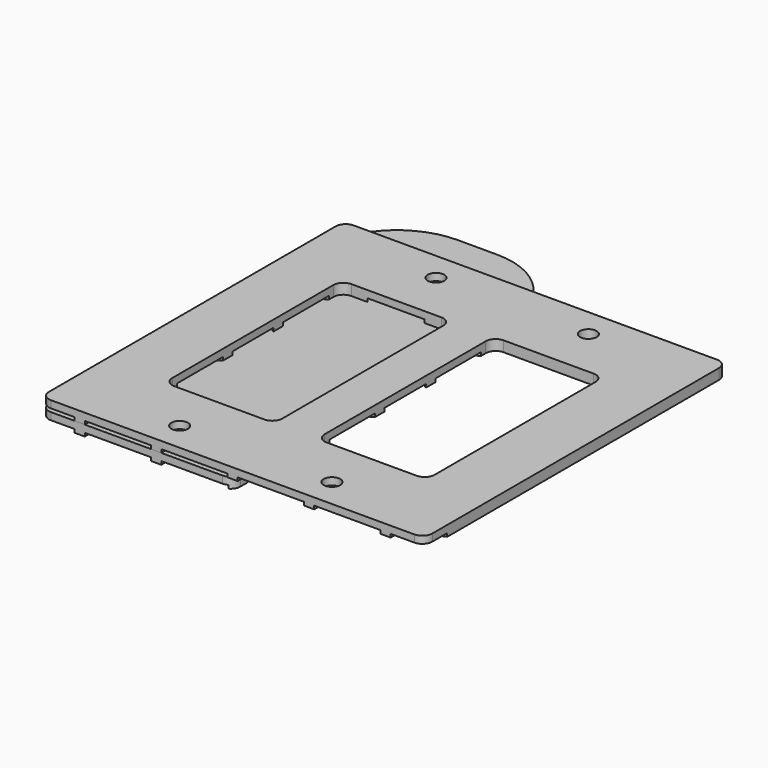
from build123d import *

# Parameters (mm, degrees)
F0_W     = 57.9
F0_H     = 114.3
F0_R     = 2.5
F0_W_2   = 33.2
F0_H_2   = 66.8
F1_DEPTH = 3.175
F2_R     = 2.5
F3_DEPTH = 3.175
F4_R     = 3
F4_2_R   = 3
F7_DEPTH = 1
F8_DEPTH = 4.175


# Not quite as in the source:
# - a length typed as a fraction of an inch, garbled in the dataset ("3 / 203.2 mm" for 3/8 in), is restored


with BuildPart() as f1:
    # F0 (on Top) → F1 (new body)
    with BuildSketch(Plane.XY):
        with Locations((-28.95, 0)):
            Rectangle(F0_W, F0_H)
        with Locations((-23, -48.4)):
            Circle(F0_R, mode=Mode.SUBTRACT)
        with Locations((-23, 0)):
            Rectangle(F0_W_2, F0_H_2, mode=Mode.SUBTRACT)
        with Locations((-23, 48.4)):
            Circle(F0_R, mode=Mode.SUBTRACT)
    extrude(amount=F1_DEPTH)

    # F4
    f4_edges = [f1.edges().sort_by_distance(p)[0] for p in [
        (-57.9, 57.15, 1.5875),
        (-57.9, -57.15, 1.5875),
        (-39.6, 33.4, 1.5875),
        (-39.6, -33.4, 1.5875),
        (-6.4, -33.4, 1.5875),
        (-6.4, 33.4, 1.5875),
    ]]
    fillet(f4_edges, radius=F4_R)

    # F5: F1 across face


with BuildPart() as f3:
    # F2 (on Top) → F3 (new body)
    with BuildSketch(Plane.XY):
        with BuildLine():
            ThreePointArc((-34.9, 71.4), (-51.1634559673, 64.6634559673), (-57.9, 48.4))
            Line((-57.9, 48.4), (-57.9, -57.15))
            Line((-57.9, -57.15), (0, -57.15))
            Line((0, -57.15), (0, 48.4))
            ThreePointArc((0, 48.4), (-6.7365440327, 64.6634559673), (-23, 71.4))
            Line((-23, 71.4), (-34.9, 71.4))
        make_face()
        with Locations((-23, -48.4)):
            Circle(F2_R, mode=Mode.SUBTRACT)
        with Locations((-23, 48.4)):
            Circle(F2_R, mode=Mode.SUBTRACT)
    extrude(amount=-F3_DEPTH)

    # F4#2
    f4_2_edges = [f3.edges().sort_by_distance(p)[0] for p in [
        (0, -57.15, -1.5875),
        (-57.9, -57.15, -1.5875),
    ]]
    fillet(f4_2_edges, radius=F4_2_R)

    # F6 (on face) → F7 (cut)
    with BuildSketch(Plane(origin=(0, 0, -3.175), x_dir=(1, 0, 0), z_dir=(0, 0, -1))):
        Polygon((57.735026919, 71.5470053838), (47.735026919, 65.7735026919), (47.735026919, 54.2264973081), (57.735026919, 48.4529946162), (67.735026919, 54.2264973081), (67.735026919, 65.7735026919), align=None)
        Polygon((36.1880215352, 45.7735026919), (36.1880215352, 34.2264973081), (46.1880215352, 28.4529946162), (56.1880215352, 34.2264973081), (56.1880215352, 45.7735026919), (46.1880215352, 51.5470053838), align=None)
        Polygon((24.6410161514, 25.7735026919), (24.6410161514, 14.2264973081), (34.6410161514, 8.4529946162), (44.6410161514, 14.2264973081), (44.6410161514, 25.7735026919), (34.6410161514, 31.5470053838), align=None)
        Polygon((13.0940107676, 5.7735026919), (13.0940107676, -5.7735026919), (23.0940107676, -11.5470053838), (33.0940107676, -5.7735026919), (33.0940107676, 5.7735026919), (23.0940107676, 11.5470053838), align=None)
        Polygon((1.5470053838, -14.2264973081), (1.5470053838, -25.7735026919), (11.5470053838, -31.5470053838), (21.5470053838, -25.7735026919), (21.5470053838, -14.2264973081), (11.5470053838, -8.4529946162), align=None)
        Polygon((24.6410161514, 65.7735026919), (24.6410161514, 54.2264973081), (34.6410161514, 48.4529946162), (44.6410161514, 54.2264973081), (44.6410161514, 65.7735026919), (34.6410161514, 71.5470053838), align=None)
        Polygon((13.0940107676, 45.7735026919), (13.0940107676, 34.2264973081), (23.0940107676, 28.4529946162), (33.0940107676, 34.2264973081), (33.0940107676, 45.7735026919), (23.0940107676, 51.5470053838), align=None)
        Polygon((1.5470053838, 25.7735026919), (1.5470053838, 14.2264973081), (11.5470053838, 8.4529946162), (21.5470053838, 14.2264973081), (21.5470053838, 25.7735026919), (11.5470053838, 31.5470053838), align=None)
        Polygon((-10, 5.7735026919), (-10, -5.7735026919), (0, -11.5470053838), (10, -5.7735026919), (10, 5.7735026919), (0, 11.5470053838), align=None)
        Polygon((-21.5470053838, -14.2264973081), (-21.5470053838, -25.7735026919), (-11.5470053838, -31.5470053838), (-1.5470053838, -25.7735026919), (-1.5470053838, -14.2264973081), (-11.5470053838, -8.4529946162), align=None)
        Polygon((1.5470053838, 65.7735026919), (1.5470053838, 54.2264973081), (11.5470053838, 48.4529946162), (21.5470053838, 54.2264973081), (21.5470053838, 65.7735026919), (11.5470053838, 71.5470053838), align=None)
        Polygon((-10, 45.7735026919), (-10, 34.2264973081), (0, 28.4529946162), (10, 34.2264973081), (10, 45.7735026919), (0, 51.5470053838), align=None)
        Polygon((-21.5470053838, 25.7735026919), (-21.5470053838, 14.2264973081), (-11.5470053838, 8.4529946162), (-1.5470053838, 14.2264973081), (-1.5470053838, 25.7735026919), (-11.5470053838, 31.5470053838), align=None)
        Polygon((-33.0940107676, 5.7735026919), (-33.0940107676, -5.7735026919), (-23.0940107676, -11.5470053838), (-13.0940107676, -5.7735026919), (-13.0940107676, 5.7735026919), (-23.0940107676, 11.5470053838), align=None)
        Polygon((-44.6410161514, -14.2264973081), (-44.6410161514, -25.7735026919), (-34.6410161514, -31.5470053838), (-24.6410161514, -25.7735026919), (-24.6410161514, -14.2264973081), (-34.6410161514, -8.4529946162), align=None)
        Polygon((-10, -34.2264973081), (-10, -45.7735026919), (0, -51.5470053838), (10, -45.7735026919), (10, -34.2264973081), (0, -28.4529946162), align=None)
        Polygon((-21.5470053838, -54.2264973081), (-21.5470053838, -65.7735026919), (-11.5470053838, -71.5470053838), (-1.5470053838, -65.7735026919), (-1.5470053838, -54.2264973081), (-11.5470053838, -48.4529946162), align=None)
        Polygon((-33.0940107676, -34.2264973081), (-33.0940107676, -45.7735026919), (-23.0940107676, -51.5470053838), (-13.0940107676, -45.7735026919), (-13.0940107676, -34.2264973081), (-23.0940107676, -28.4529946162), align=None)
        Polygon((-44.6410161514, -54.2264973081), (-44.6410161514, -65.7735026919), (-34.6410161514, -71.5470053838), (-24.6410161514, -65.7735026919), (-24.6410161514, -54.2264973081), (-34.6410161514, -48.4529946162), align=None)
        Polygon((-56.1880215352, -34.2264973081), (-56.1880215352, -45.7735026919), (-46.1880215352, -51.5470053838), (-36.1880215352, -45.7735026919), (-36.1880215352, -34.2264973081), (-46.1880215352, -28.4529946162), align=None)
        Polygon((-67.735026919, -54.2264973081), (-67.735026919, -65.7735026919), (-57.735026919, -71.5470053838), (-47.735026919, -65.7735026919), (-47.735026919, -54.2264973081), (-57.735026919, -48.4529946162), align=None)
        Polygon((-21.5470053838, 65.7735026919), (-21.5470053838, 54.2264973081), (-11.5470053838, 48.4529946162), (-1.5470053838, 54.2264973081), (-1.5470053838, 65.7735026919), (-11.5470053838, 71.5470053838), align=None)
        Polygon((-33.0940107676, 45.7735026919), (-33.0940107676, 34.2264973081), (-23.0940107676, 28.4529946162), (-13.0940107676, 34.2264973081), (-13.0940107676, 45.7735026919), (-23.0940107676, 51.5470053838), align=None)
        Polygon((-44.6410161514, 25.7735026919), (-44.6410161514, 14.2264973081), (-34.6410161514, 8.4529946162), (-24.6410161514, 14.2264973081), (-24.6410161514, 25.7735026919), (-34.6410161514, 31.5470053838), align=None)
        Polygon((-56.1880215352, 5.7735026919), (-56.1880215352, -5.7735026919), (-46.1880215352, -11.5470053838), (-36.1880215352, -5.7735026919), (-36.1880215352, 5.7735026919), (-46.1880215352, 11.5470053838), align=None)
        Polygon((-67.735026919, -14.2264973081), (-67.735026919, -25.7735026919), (-57.735026919, -31.5470053838), (-47.735026919, -25.7735026919), (-47.735026919, -14.2264973081), (-57.735026919, -8.4529946162), align=None)
        Polygon((-79.2820323028, -34.2264973081), (-79.2820323028, -45.7735026919), (-69.2820323028, -51.5470053838), (-59.2820323028, -45.7735026919), (-59.2820323028, -34.2264973081), (-69.2820323028, -28.4529946162), align=None)
        Polygon((-90.8290376865, -54.2264973081), (-90.8290376865, -65.7735026919), (-80.8290376865, -71.5470053838), (-70.8290376865, -65.7735026919), (-70.8290376865, -54.2264973081), (-80.8290376865, -48.4529946162), align=None)
        Polygon((-44.6410161514, 65.7735026919), (-44.6410161514, 54.2264973081), (-34.6410161514, 48.4529946162), (-24.6410161514, 54.2264973081), (-24.6410161514, 65.7735026919), (-34.6410161514, 71.5470053838), align=None)
        Polygon((-56.1880215352, 45.7735026919), (-56.1880215352, 34.2264973081), (-46.1880215352, 28.4529946162), (-36.1880215352, 34.2264973081), (-36.1880215352, 45.7735026919), (-46.1880215352, 51.5470053838), align=None)
        Polygon((-67.735026919, 25.7735026919), (-67.735026919, 14.2264973081), (-57.735026919, 8.4529946162), (-47.735026919, 14.2264973081), (-47.735026919, 25.7735026919), (-57.735026919, 31.5470053838), align=None)
        Polygon((-79.2820323028, 5.7735026919), (-79.2820323028, -5.7735026919), (-69.2820323028, -11.5470053838), (-59.2820323028, -5.7735026919), (-59.2820323028, 5.7735026919), (-69.2820323028, 11.5470053838), align=None)
        Polygon((-90.8290376865, -14.2264973081), (-90.8290376865, -25.7735026919), (-80.8290376865, -31.5470053838), (-70.8290376865, -25.7735026919), (-70.8290376865, -14.2264973081), (-80.8290376865, -8.4529946162), align=None)
        Polygon((-102.3760430703, -34.2264973081), (-102.3760430703, -45.7735026919), (-92.3760430703, -51.5470053838), (-82.3760430703, -45.7735026919), (-82.3760430703, -34.2264973081), (-92.3760430703, -28.4529946162), align=None)
        Polygon((-113.9230484541, -54.2264973081), (-113.9230484541, -65.7735026919), (-103.9230484541, -71.5470053838), (-93.9230484541, -65.7735026919), (-93.9230484541, -54.2264973081), (-103.9230484541, -48.4529946162), align=None)
        Polygon((-67.735026919, 65.7735026919), (-67.735026919, 54.2264973081), (-57.735026919, 48.4529946162), (-47.735026919, 54.2264973081), (-47.735026919, 65.7735026919), (-57.735026919, 71.5470053838), align=None)
        Polygon((-79.2820323028, 45.7735026919), (-79.2820323028, 34.2264973081), (-69.2820323028, 28.4529946162), (-59.2820323028, 34.2264973081), (-59.2820323028, 45.7735026919), (-69.2820323028, 51.5470053838), align=None)
        Polygon((-90.8290376865, 25.7735026919), (-90.8290376865, 14.2264973081), (-80.8290376865, 8.4529946162), (-70.8290376865, 14.2264973081), (-70.8290376865, 25.7735026919), (-80.8290376865, 31.5470053838), align=None)
        Polygon((-102.3760430703, 5.7735026919), (-102.3760430703, -5.7735026919), (-92.3760430703, -11.5470053838), (-82.3760430703, -5.7735026919), (-82.3760430703, 5.7735026919), (-92.3760430703, 11.5470053838), align=None)
        Polygon((-113.9230484541, -14.2264973081), (-113.9230484541, -25.7735026919), (-103.9230484541, -31.5470053838), (-93.9230484541, -25.7735026919), (-93.9230484541, -14.2264973081), (-103.9230484541, -8.4529946162), align=None)
        Polygon((-125.4700538379, -34.2264973081), (-125.4700538379, -45.7735026919), (-115.4700538379, -51.5470053838), (-105.4700538379, -45.7735026919), (-105.4700538379, -34.2264973081), (-115.4700538379, -28.4529946162), align=None)
        Polygon((-137.0170592217, -54.2264973081), (-137.0170592217, -65.7735026919), (-127.0170592217, -71.5470053838), (-117.0170592217, -65.7735026919), (-117.0170592217, -54.2264973081), (-127.0170592217, -48.4529946162), align=None)
    extrude(amount=-F7_DEPTH, mode=Mode.SUBTRACT)


with BuildPart() as f1_1:
    add(f1.part)
    add(f1.part.mirror(Plane(origin=(0, 0, 1.5875), x_dir=(0, 1, 0), z_dir=(1, 0, 0))))

    # F6 (on face) → F8 (cut)
    with BuildSketch(Plane(origin=(0, 0, -3.175), x_dir=(1, 0, 0), z_dir=(0, 0, -1))):
        Polygon((57.735026919, 71.5470053838), (47.735026919, 65.7735026919), (47.735026919, 54.2264973081), (57.735026919, 48.4529946162), (67.735026919, 54.2264973081), (67.735026919, 65.7735026919), align=None)
        Polygon((36.1880215352, 45.7735026919), (36.1880215352, 34.2264973081), (46.1880215352, 28.4529946162), (56.1880215352, 34.2264973081), (56.1880215352, 45.7735026919), (46.1880215352, 51.5470053838), align=None)
        Polygon((24.6410161514, 25.7735026919), (24.6410161514, 14.2264973081), (34.6410161514, 8.4529946162), (44.6410161514, 14.2264973081), (44.6410161514, 25.7735026919), (34.6410161514, 31.5470053838), align=None)
        Polygon((13.0940107676, 5.7735026919), (13.0940107676, -5.7735026919), (23.0940107676, -11.5470053838), (33.0940107676, -5.7735026919), (33.0940107676, 5.7735026919), (23.0940107676, 11.5470053838), align=None)
        Polygon((1.5470053838, -14.2264973081), (1.5470053838, -25.7735026919), (11.5470053838, -31.5470053838), (21.5470053838, -25.7735026919), (21.5470053838, -14.2264973081), (11.5470053838, -8.4529946162), align=None)
        Polygon((24.6410161514, 65.7735026919), (24.6410161514, 54.2264973081), (34.6410161514, 48.4529946162), (44.6410161514, 54.2264973081), (44.6410161514, 65.7735026919), (34.6410161514, 71.5470053838), align=None)
        Polygon((13.0940107676, 45.7735026919), (13.0940107676, 34.2264973081), (23.0940107676, 28.4529946162), (33.0940107676, 34.2264973081), (33.0940107676, 45.7735026919), (23.0940107676, 51.5470053838), align=None)
        Polygon((1.5470053838, 25.7735026919), (1.5470053838, 14.2264973081), (11.5470053838, 8.4529946162), (21.5470053838, 14.2264973081), (21.5470053838, 25.7735026919), (11.5470053838, 31.5470053838), align=None)
        Polygon((-10, 5.7735026919), (-10, -5.7735026919), (0, -11.5470053838), (10, -5.7735026919), (10, 5.7735026919), (0, 11.5470053838), align=None)
        Polygon((-21.5470053838, -14.2264973081), (-21.5470053838, -25.7735026919), (-11.5470053838, -31.5470053838), (-1.5470053838, -25.7735026919), (-1.5470053838, -14.2264973081), (-11.5470053838, -8.4529946162), align=None)
        Polygon((1.5470053838, 65.7735026919), (1.5470053838, 54.2264973081), (11.5470053838, 48.4529946162), (21.5470053838, 54.2264973081), (21.5470053838, 65.7735026919), (11.5470053838, 71.5470053838), align=None)
        Polygon((-10, 45.7735026919), (-10, 34.2264973081), (0, 28.4529946162), (10, 34.2264973081), (10, 45.7735026919), (0, 51.5470053838), align=None)
        Polygon((-21.5470053838, 25.7735026919), (-21.5470053838, 14.2264973081), (-11.5470053838, 8.4529946162), (-1.5470053838, 14.2264973081), (-1.5470053838, 25.7735026919), (-11.5470053838, 31.5470053838), align=None)
        Polygon((-33.0940107676, 5.7735026919), (-33.0940107676, -5.7735026919), (-23.0940107676, -11.5470053838), (-13.0940107676, -5.7735026919), (-13.0940107676, 5.7735026919), (-23.0940107676, 11.5470053838), align=None)
        Polygon((-44.6410161514, -14.2264973081), (-44.6410161514, -25.7735026919), (-34.6410161514, -31.5470053838), (-24.6410161514, -25.7735026919), (-24.6410161514, -14.2264973081), (-34.6410161514, -8.4529946162), align=None)
        Polygon((-10, -34.2264973081), (-10, -45.7735026919), (0, -51.5470053838), (10, -45.7735026919), (10, -34.2264973081), (0, -28.4529946162), align=None)
        Polygon((-21.5470053838, -54.2264973081), (-21.5470053838, -65.7735026919), (-11.5470053838, -71.5470053838), (-1.5470053838, -65.7735026919), (-1.5470053838, -54.2264973081), (-11.5470053838, -48.4529946162), align=None)
        Polygon((-33.0940107676, -34.2264973081), (-33.0940107676, -45.7735026919), (-23.0940107676, -51.5470053838), (-13.0940107676, -45.7735026919), (-13.0940107676, -34.2264973081), (-23.0940107676, -28.4529946162), align=None)
        Polygon((-44.6410161514, -54.2264973081), (-44.6410161514, -65.7735026919), (-34.6410161514, -71.5470053838), (-24.6410161514, -65.7735026919), (-24.6410161514, -54.2264973081), (-34.6410161514, -48.4529946162), align=None)
        Polygon((-56.1880215352, -34.2264973081), (-56.1880215352, -45.7735026919), (-46.1880215352, -51.5470053838), (-36.1880215352, -45.7735026919), (-36.1880215352, -34.2264973081), (-46.1880215352, -28.4529946162), align=None)
        Polygon((-67.735026919, -54.2264973081), (-67.735026919, -65.7735026919), (-57.735026919, -71.5470053838), (-47.735026919, -65.7735026919), (-47.735026919, -54.2264973081), (-57.735026919, -48.4529946162), align=None)
        Polygon((-21.5470053838, 65.7735026919), (-21.5470053838, 54.2264973081), (-11.5470053838, 48.4529946162), (-1.5470053838, 54.2264973081), (-1.5470053838, 65.7735026919), (-11.5470053838, 71.5470053838), align=None)
        Polygon((-33.0940107676, 45.7735026919), (-33.0940107676, 34.2264973081), (-23.0940107676, 28.4529946162), (-13.0940107676, 34.2264973081), (-13.0940107676, 45.7735026919), (-23.0940107676, 51.5470053838), align=None)
        Polygon((-44.6410161514, 25.7735026919), (-44.6410161514, 14.2264973081), (-34.6410161514, 8.4529946162), (-24.6410161514, 14.2264973081), (-24.6410161514, 25.7735026919), (-34.6410161514, 31.5470053838), align=None)
        Polygon((-56.1880215352, 5.7735026919), (-56.1880215352, -5.7735026919), (-46.1880215352, -11.5470053838), (-36.1880215352, -5.7735026919), (-36.1880215352, 5.7735026919), (-46.1880215352, 11.5470053838), align=None)
        Polygon((-67.735026919, -14.2264973081), (-67.735026919, -25.7735026919), (-57.735026919, -31.5470053838), (-47.735026919, -25.7735026919), (-47.735026919, -14.2264973081), (-57.735026919, -8.4529946162), align=None)
        Polygon((-79.2820323028, -34.2264973081), (-79.2820323028, -45.7735026919), (-69.2820323028, -51.5470053838), (-59.2820323028, -45.7735026919), (-59.2820323028, -34.2264973081), (-69.2820323028, -28.4529946162), align=None)
        Polygon((-90.8290376865, -54.2264973081), (-90.8290376865, -65.7735026919), (-80.8290376865, -71.5470053838), (-70.8290376865, -65.7735026919), (-70.8290376865, -54.2264973081), (-80.8290376865, -48.4529946162), align=None)
        Polygon((-44.6410161514, 65.7735026919), (-44.6410161514, 54.2264973081), (-34.6410161514, 48.4529946162), (-24.6410161514, 54.2264973081), (-24.6410161514, 65.7735026919), (-34.6410161514, 71.5470053838), align=None)
        Polygon((-56.1880215352, 45.7735026919), (-56.1880215352, 34.2264973081), (-46.1880215352, 28.4529946162), (-36.1880215352, 34.2264973081), (-36.1880215352, 45.7735026919), (-46.1880215352, 51.5470053838), align=None)
        Polygon((-67.735026919, 25.7735026919), (-67.735026919, 14.2264973081), (-57.735026919, 8.4529946162), (-47.735026919, 14.2264973081), (-47.735026919, 25.7735026919), (-57.735026919, 31.5470053838), align=None)
        Polygon((-79.2820323028, 5.7735026919), (-79.2820323028, -5.7735026919), (-69.2820323028, -11.5470053838), (-59.2820323028, -5.7735026919), (-59.2820323028, 5.7735026919), (-69.2820323028, 11.5470053838), align=None)
        Polygon((-90.8290376865, -14.2264973081), (-90.8290376865, -25.7735026919), (-80.8290376865, -31.5470053838), (-70.8290376865, -25.7735026919), (-70.8290376865, -14.2264973081), (-80.8290376865, -8.4529946162), align=None)
        Polygon((-102.3760430703, -34.2264973081), (-102.3760430703, -45.7735026919), (-92.3760430703, -51.5470053838), (-82.3760430703, -45.7735026919), (-82.3760430703, -34.2264973081), (-92.3760430703, -28.4529946162), align=None)
        Polygon((-113.9230484541, -54.2264973081), (-113.9230484541, -65.7735026919), (-103.9230484541, -71.5470053838), (-93.9230484541, -65.7735026919), (-93.9230484541, -54.2264973081), (-103.9230484541, -48.4529946162), align=None)
        Polygon((-67.735026919, 65.7735026919), (-67.735026919, 54.2264973081), (-57.735026919, 48.4529946162), (-47.735026919, 54.2264973081), (-47.735026919, 65.7735026919), (-57.735026919, 71.5470053838), align=None)
        Polygon((-79.2820323028, 45.7735026919), (-79.2820323028, 34.2264973081), (-69.2820323028, 28.4529946162), (-59.2820323028, 34.2264973081), (-59.2820323028, 45.7735026919), (-69.2820323028, 51.5470053838), align=None)
        Polygon((-90.8290376865, 25.7735026919), (-90.8290376865, 14.2264973081), (-80.8290376865, 8.4529946162), (-70.8290376865, 14.2264973081), (-70.8290376865, 25.7735026919), (-80.8290376865, 31.5470053838), align=None)
        Polygon((-102.3760430703, 5.7735026919), (-102.3760430703, -5.7735026919), (-92.3760430703, -11.5470053838), (-82.3760430703, -5.7735026919), (-82.3760430703, 5.7735026919), (-92.3760430703, 11.5470053838), align=None)
        Polygon((-113.9230484541, -14.2264973081), (-113.9230484541, -25.7735026919), (-103.9230484541, -31.5470053838), (-93.9230484541, -25.7735026919), (-93.9230484541, -14.2264973081), (-103.9230484541, -8.4529946162), align=None)
        Polygon((-125.4700538379, -34.2264973081), (-125.4700538379, -45.7735026919), (-115.4700538379, -51.5470053838), (-105.4700538379, -45.7735026919), (-105.4700538379, -34.2264973081), (-115.4700538379, -28.4529946162), align=None)
        Polygon((-137.0170592217, -54.2264973081), (-137.0170592217, -65.7735026919), (-127.0170592217, -71.5470053838), (-117.0170592217, -65.7735026919), (-117.0170592217, -54.2264973081), (-127.0170592217, -48.4529946162), align=None)
    extrude(amount=-F8_DEPTH, mode=Mode.SUBTRACT)


solid = Compound([f3.part, f1_1.part])
